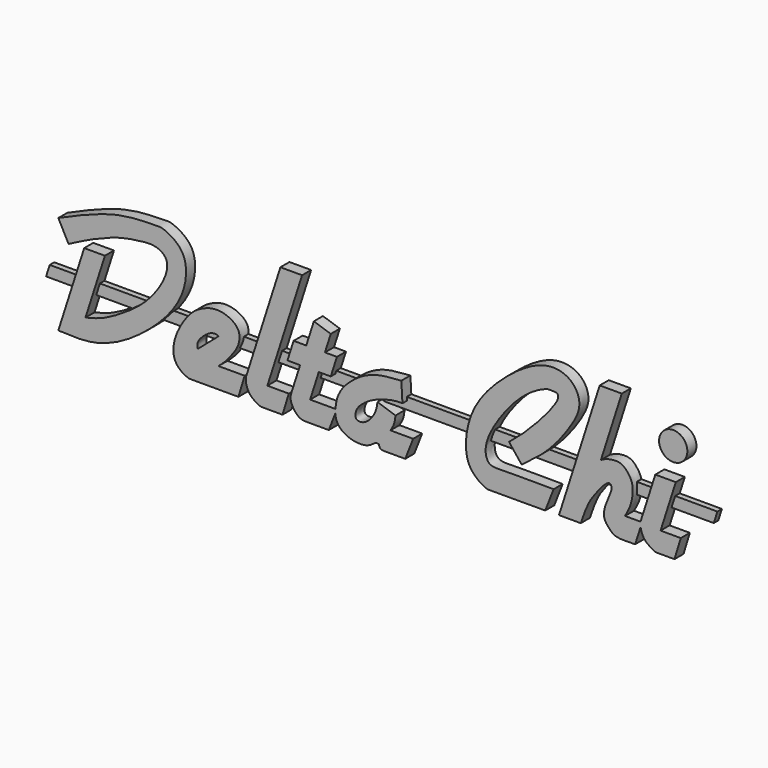
from build123d import *

# Parameters (mm, degrees)
F1_DEPTH = 1.27
F0_R     = 1.5843769343
F4_DEPTH = 0.635
F5_DEPTH = 0.635


with BuildPart() as f1:
    # F0 (on Front) → F1 (new body)
    with BuildSketch(Plane.XZ):
        with BuildLine():
            Line((11.5583368814, 2.9581922572), (9.238501317, 2.9581922572))
            Line((9.238501317, 2.9581922572), (6.3397404738, -6.112227682))
            add(Edge.make_bspline(
                [(6.3397404738, -6.112227682), (7.4441484176, -6.1544100754), (11.509628416, -6.5846275927), (17.9109968749, -1.8961025658), (20.4928464292, 1.9472420269), (20.817384408, 5.0494202074), (19.9129921351, 6.8743066297), (17.9478352073, 7.8694620029), (17.2190347579, 7.7492274241), (12.7951441267, 7.8669975564), (8.7299015863, 6.0410147356), (6.3397404738, 4.9838235872)],
                knots=[0, 0, 0, 0, 0.1269238793, 0.2901043112, 0.4152988438, 0.5132554474, 0.5948026218, 0.6765960194, 0.7255936362, 0.8411976173, 1, 1, 1, 1], degree=3))
            Line((6.3397404738, 4.9838235872), (7.4859545566, 2.7952580713))
            add(Edge.make_bspline(
                [(7.4859545566, 2.7952580713), (8.2236601536, 3.1805826506), (9.8172231795, 4.01295741), (12.9982791172, 5.3295282857), (15.1573844049, 5.6487607974), (17.2331239985, 5.9184782824), (18.7492748451, 4.9172200411), (18.3797124669, 2.7652905985), (16.3268092986, -0.1702231309), (13.6664187703, -2.0050802173), (11.597224487, -3.2305518663), (10.2401798172, -3.6615941397), (9.3834213912, -3.8472663146)],
                knots=[0, 0, 0, 0, 0.1035319794, 0.2210262779, 0.3162776823, 0.4065161292, 0.4835580268, 0.5705705005, 0.6913426498, 0.8065191141, 0.9033937832, 1, 1, 1, 1], degree=3))
            Line((9.3834213912, -3.8472663146), (11.5583368814, 2.9581922572))
        make_face()
    extrude(amount=F1_DEPTH)


with BuildPart() as f1b:
    # F0 (on Front) → F1, piece 2 (new body)
    with BuildSketch(Plane.XZ):
        with BuildLine():
            Line((27.2133555263, -3.7849494256), (24.2806579918, -3.7849494256))
            add(Edge.make_bspline(
                [(20.934375003, -6.0972687788), (20.6237746916, -5.9553557041), (19.9688638955, -5.656127399), (19.0898046825, -4.5438356782), (19.3260874159, -2.3470660746), (20.6114467926, -0.1690673469), (21.7037779099, 0.9830999374), (23.5887847531, 1.8522113729), (25.3229288137, 1.5984111399), (26.7458523187, 0.6140665528), (26.6181462164, -1.0302522959), (25.8346105799, -2.1262963733), (25.1208132675, -3.0535019221), (24.5582846254, -3.5432449289), (24.2806579918, -3.7849494256)],
                knots=[0, 0, 0, 0, 0.0683310471, 0.1440782214, 0.2416800374, 0.3481729944, 0.4329900458, 0.5268903062, 0.6150450793, 0.6982655618, 0.7790626002, 0.8570259985, 0.929437565, 1, 1, 1, 1], degree=3))
            Line((20.934375003, -6.0972687788), (26.5177804977, -6.0972687788))
            Line((26.5177804977, -6.0972687788), (27.2133555263, -3.7849494256))
        make_face()
        with BuildLine():
            add(Edge.make_bspline(
                [(21.9683405012, -2.8449825477), (22.739112998, -2.1807390925), (23.5098854949, -1.5164956373), (24.2806579918, -0.8522521821)],
                knots=[0, 0, 0, 0, 3.0525049529, 3.0525049529, 3.0525049529, 3.0525049529], degree=3))
            add(Edge.make_bspline(
                [(21.9683405012, -2.8449825477), (21.9220461308, -2.6323953166), (21.8022425221, -2.1277051513), (22.9283600883, -1.0010714427), (23.7222803055, -0.6785461743), (24.1428096339, -0.7291242349), (24.2806579918, -0.8522521821)],
                knots=[0, 0, 0, 0, 0.2196054864, 0.550181783, 0.8035281405, 1, 1, 1, 1], degree=3))
        make_face(mode=Mode.SUBTRACT)
    extrude(amount=F1_DEPTH)


with BuildPart() as f1c:
    # F0 (on Front) → F1, piece 3 (new body)
    with BuildSketch(Plane.XZ):
        with BuildLine():
            Line((29.7624055112, -3.9401776428), (33.6480308079, 8.2182083279))
            Line((33.6480308079, 8.2182083279), (31.2219001353, 8.2182083279))
            Line((31.2219001353, 8.2182083279), (27.395882284, -3.7536618897))
            add(Edge.make_bspline(
                [(27.395882284, -3.7536618897), (27.3626673092, -3.9107859252), (27.2830365237, -4.2882497343), (27.6099014615, -5.2582507547), (28.1522354832, -5.7998826823), (28.6683587416, -6.0880579287), (28.9955866819, -6.2549276858), (29.1592962131, -6.2536320454)],
                knots=[0, 0, 0, 0, 0.1777965485, 0.4222191522, 0.6373839909, 0.8255478489, 1, 1, 1, 1], degree=3))
            Line((29.1592962131, -6.2536320454), (31.4544699177, -6.2536320454))
            Line((31.4544699177, -6.2536320454), (32.1586950704, -3.9401776428))
            Line((32.1586950704, -3.9401776428), (29.7624055112, -3.9401776428))
        make_face()
    extrude(amount=F1_DEPTH)


with BuildPart() as f1d:
    # F0 (on Front) → F1, piece 4 (new body)
    with BuildSketch(Plane.XZ):
        with BuildLine():
            Line((34.1174524835, 1.4392599511), (32.6996871635, 1.4392599511))
            Line((32.6996871635, 1.4392599511), (32.0095790109, -0.7201354202))
            Line((32.0095790109, -0.7201354202), (33.427344331, -0.7201354202))
            Line((33.427344331, -0.7201354202), (32.3894061148, -3.9679147303))
            add(Edge.make_bspline(
                [(32.3894061148, -3.9679147303), (32.3539821517, -4.2074069235), (32.3077429237, -4.5448398513), (32.8789397145, -5.6686856111), (33.6315587034, -6.0905655252), (34.0119533579, -6.0804787938), (34.1916170495, -6.0811438617)],
                knots=[0, 0, 0, 0, 0.2197878812, 0.5298954364, 0.7910428436, 1, 1, 1, 1], degree=3))
            Line((34.1916170495, -6.0811438617), (36.6396096127, -6.0811438617))
            Line((36.6396096127, -6.0811438617), (37.3817411468, -4.1773119798))
            add(Edge.make_bspline(
                [(37.390926157, -3.7552919632), (37.3804727481, -3.896675323), (37.3761926951, -4.0379928618), (37.3817411468, -4.1773119798)],
                knots=[0.5705734468, 0.5705734468, 0.5705734468, 0.5705734468, 0.6009630692, 0.6009630692, 0.6009630692, 0.6009630692], degree=3))
            Line((37.390926157, -3.7552919632), (34.5505749426, -3.7552919632))
            Line((34.5505749426, -3.7552919632), (35.5205623301, -0.7201354202))
            Line((35.5205623301, -0.7201354202), (36.8627270243, -0.7201354202))
            Line((36.8627270243, -0.7201354202), (37.5528351768, 1.4392599511))
            Line((37.5528351768, 1.4392599511), (36.2106704826, 1.4392599511))
            Line((36.2106704826, 1.4392599511), (36.8627270243, 3.4795892425))
            Line((36.8627270243, 3.4795892425), (34.9704111173, 4.10822556))
            Line((34.9704111173, 4.10822556), (34.1174524835, 1.4392599511))
        make_face()
        with BuildLine():
            add(Edge.make_bspline(
                [(37.390926157, -3.7552919632), (37.3804727481, -3.896675323), (37.3761926951, -4.0379928618), (37.3817411468, -4.1773119798)],
                knots=[0.5705734468, 0.5705734468, 0.5705734468, 0.5705734468, 0.6009630692, 0.6009630692, 0.6009630692, 0.6009630692], degree=3))
            add(Edge.make_bspline(
                [(37.3817411468, -4.1773119798), (37.392328196, -4.4431480099), (37.5312347254, -5.2176693669), (38.7220219736, -6.236897387), (40.8587848965, -6.4300522573), (41.5571529811, -5.8736297488), (41.8619178236, -5.6308093481)],
                knots=[0.6009630692, 0.6009630692, 0.6009630692, 0.6009630692, 0.6589497741, 0.7746633228, 0.9016640387, 1, 1, 1, 1], degree=3))
            Line((41.8619178236, -5.6308093481), (42.2533527017, -5.6308093481))
            add(Edge.make_bspline(
                [(42.2533527017, -5.6308093481), (42.2675923832, -5.7180727897), (42.2968327159, -5.8972630384), (42.4875444347, -6.1218789339), (42.8100095232, -6.1339937311), (42.8472571075, -6.1338087544)],
                knots=[0, 0, 0, 0, 0.2963318136, 0.608499623, 0.9364444921, 0.9364444921, 0.9364444921, 0.9364444921], degree=3))
            Line((42.8472571075, -6.1338087544), (45.2066808939, -6.1332210898))
            Line((45.2066808939, -6.1332210898), (46.0903713247, -3.8662401858))
            Line((46.0903713247, -3.8662401858), (43.5422138314, -3.8662401858))
            add(Edge.make_bspline(
                [(43.5422138314, -3.8662401858), (43.6434718788, -3.7248078476), (43.955566276, -3.202149882), (44.0373991751, -2.8050103574), (44.1166646779, -2.2105039097)],
                knots=[0, 0, 0, 0, 0.4355065819, 1, 1, 1, 1], degree=3))
            Line((44.1166646779, -2.2105039097), (42.0921580655, -1.5379532131))
            add(Edge.make_bspline(
                [(44.8928326368, -0.7567268331), (44.4289408624, -0.7455486339), (44.334726943, -0.7630375022), (43.4964447415, -0.834955831), (41.5388628103, -1.390907753), (40.090989198, -2.4696041182), (39.6410756327, -3.1901824428), (39.5414913588, -4.1442095313), (40.8415428068, -4.1903256763), (41.961217304, -2.6601737366), (42.0533731488, -1.8780982635), (42.0921580655, -1.5379532131)],
                knots=[0, 0, 0, 0, 0.0840952071, 0.1697088013, 0.3216193436, 0.4624728163, 0.5586747749, 0.6467834882, 0.7479812036, 0.8890732838, 1, 1, 1, 1], degree=3))
            Line((44.8928326368, -0.7567268331), (44.7697676718, 1.432727091))
            add(Edge.make_bspline(
                [(44.7697676718, 1.432727091), (43.7008223192, 1.3640593706), (41.648313579, 1.232208761), (39.3385119054, -0.1260462045), (37.7342234004, -1.8446619748), (37.4613840971, -3.0431148695), (37.3978194533, -3.6620594683), (37.390926157, -3.7552919632)],
                knots=[0, 0, 0, 0, 0.1578260616, 0.3030457732, 0.4375753345, 0.5505336039, 0.5705734468, 0.5705734468, 0.5705734468, 0.5705734468], degree=3))
        make_face()
    extrude(amount=F1_DEPTH)


with BuildPart() as f1e:
    # F0 (on Front) → F1, piece 5 (new body)
    with BuildSketch(Plane.XZ):
        with BuildLine():
            add(Edge.make_bspline(
                [(56.8344220519, -0.6727006403), (57.536092901, -0.0985210669), (58.981812623, 1.0845161568), (61.4522683866, 3.8814649904), (61.4833894251, 4.0843152011), (62.367054076, 5.1445088036), (62.3973875748, 5.9770064502), (61.5374535241, 5.9113985648), (61.1907722065, 6.0054789768), (59.3549616868, 5.219553597), (56.8962905087, 3.0575959186), (54.476325238, -0.5239799869), (54.0840321515, -2.5259321439), (54.5585012014, -3.7841258338), (56.4829070286, -3.6899333482), (59.7177449421, -3.7098362799), (61.8280459066, -3.723213362)],
                knots=[0, 0, 0, 0, 0.0930582141, 0.1917435104, 0.2179368983, 0.2792954818, 0.3217037626, 0.3653724828, 0.397525177, 0.4677311533, 0.5674134201, 0.678450431, 0.7529723589, 0.8065968651, 0.873879835, 1, 1, 1, 1], degree=3))
            Line((56.8344220519, -0.6727006403), (58.2509338856, -2.4686302058))
            add(Edge.make_bspline(
                [(58.2509338856, -2.4686302058), (58.4671273828, -2.2947364487), (58.653230403, -2.0939955812), (61.2401562782, -0.3340070928), (63.8132491254, 3.0521447417), (65.1156690008, 5.6462437526), (63.8351395983, 8.0752841997), (60.2374798056, 8.7326906295), (54.9538299971, 4.5474881989), (52.5011949099, 1.0432474754), (51.8172413088, -2.415022098), (52.3018042793, -4.9135195574), (54.0605011917, -6.0731752268), (54.5331237261, -6.1424866279), (54.5733683978, -6.1474639068), (60.2808153305, -6.1354543984), (60.8894621988, -6.1310150856)],
                knots=[0, 0, 0, 0, 0.0338861178, 0.1086849092, 0.2033726715, 0.2762020347, 0.3423872005, 0.4207228438, 0.5341164091, 0.6272992911, 0.7084751446, 0.7780444737, 0.8398677078, 0.866251273, 0.8837492923, 0.9909216554, 0.9909216554, 0.9909216554, 0.9909216554], degree=3))
            Line((60.8894621988, -6.1310150856), (61.8280459066, -3.723213362))
        make_face()
    extrude(amount=F1_DEPTH)


with BuildPart() as f1f:
    # F0 (on Front) → F1, piece 6 (new body)
    with BuildSketch(Plane.XZ):
        with BuildLine():
            Line((66.9940567642, 8.1950222574), (62.4304637313, -6.0847708955))
            Line((62.4304637313, -6.0847708955), (64.8716390133, -6.0847708955))
            add(Edge.make_bspline(
                [(64.8716390133, -6.0847708955), (64.9763642646, -5.7314444494), (65.3113821699, -4.8136837528), (65.8788110997, -3.4582361982), (66.6711638205, -2.4563300411), (67.2341715854, -1.6631813625), (68.1666941651, -0.8457293994), (68.449894567, -1.6855497607), (67.7251359557, -2.9881592018), (67.2711232708, -4.6517195726), (68.0296074984, -5.5527121429), (68.7566935376, -6.2902897156), (70.0967212544, -6.1977129943), (70.9676982654, -6.1819385307)],
                knots=[0, 0, 0, 0, 0.0940386819, 0.1947266023, 0.286033855, 0.3709752136, 0.4506078612, 0.508931595, 0.6105547438, 0.7159243693, 0.7998688722, 0.8786044105, 1, 1, 1, 1], degree=3))
            Line((70.9676982654, -6.1819385307), (71.5720379679, -4.2909184761))
            add(Edge.make_bspline(
                [(71.5710121124, -3.7578128137), (71.5441535969, -3.8975253136), (71.5336089809, -4.0521583348), (71.5670617144, -4.2631440018), (71.5720379679, -4.2909184761)],
                knots=[0.0137477144, 0.0137477144, 0.0137477144, 0.0137477144, 0.1731956127, 0.1966109127, 0.1966109127, 0.1966109127, 0.1966109127], degree=3))
            Line((71.5710121124, -3.7578128137), (69.8300384912, -3.7578128137))
            add(Edge.make_bspline(
                [(67.1309805195, 0.8867597493), (67.3340182593, 0.9992655484), (67.8150259898, 1.2657686397), (69.369655112, 1.4777996976), (70.1951225015, 0.6081433229), (70.8397112827, -0.4415409908), (70.5571540861, -2.5072653543), (70.0498844289, -3.3604386206), (69.8300384912, -3.7578128137)],
                knots=[0, 0, 0, 0, 0.1288060496, 0.3049437453, 0.4582521101, 0.6175575441, 0.8236651085, 1, 1, 1, 1], degree=3))
            Line((67.1309805195, 0.8867597493), (69.4665840894, 8.1950222574))
            Line((69.4665840894, 8.1950222574), (66.9940567642, 8.1950222574))
        make_face()
        with BuildLine():
            add(Edge.make_bspline(
                [(71.5710121124, -3.7578128137), (71.5441535969, -3.8975253136), (71.5336089809, -4.0521583348), (71.5670617144, -4.2631440018), (71.5720379679, -4.2909184761)],
                knots=[0.0137477144, 0.0137477144, 0.0137477144, 0.0137477144, 0.1731956127, 0.1966109127, 0.1966109127, 0.1966109127, 0.1966109127], degree=3))
            add(Edge.make_bspline(
                [(71.5720379679, -4.2909184761), (71.6194594312, -4.5555967542), (71.8370975302, -5.2135369306), (72.3605804566, -5.7393451035), (72.8886416365, -6.003119047), (73.1790271773, -6.2227930925), (73.341757151, -6.2215052046)],
                knots=[0.1966109127, 0.1966109127, 0.1966109127, 0.1966109127, 0.4197482157, 0.6367880894, 0.8265916848, 1, 1, 1, 1], degree=3))
            Line((73.341757151, -6.2215052046), (75.3721089563, -6.2215052046))
            Line((75.3721089563, -6.2215052046), (76.076334109, -3.908050802))
            Line((76.076334109, -3.908050802), (73.8132742946, -3.908050802))
            Line((73.8132742946, -3.908050802), (75.5176777163, 1.4251434891))
            Line((75.5176777163, 1.4251434891), (73.2231391982, 1.4251434891))
            Line((73.2231391982, 1.4251434891), (71.578343222, -3.7215350489))
            add(Edge.make_bspline(
                [(71.578343222, -3.7215350489), (71.5757749495, -3.7336843082), (71.5733278733, -3.7457666998), (71.5710121124, -3.7578128137)],
                knots=[0, 0, 0, 0, 0.0137477144, 0.0137477144, 0.0137477144, 0.0137477144], degree=3))
        make_face()
    extrude(amount=F1_DEPTH)


with BuildPart() as f1g:
    # F0 (on Front) → F1, piece 7 (new body)
    with BuildSketch(Plane.XZ):
        with Locations((75.2293908452, 4.8940147229)):
            Circle(F0_R)
    extrude(amount=F1_DEPTH)


with BuildPart() as f1_1:
    # F2: moved
    add(f1.part.moved(Location((0, 0, 1.016))))



with BuildPart() as f1b_1:
    # F2: moved
    add(f1b.part.moved(Location((0, 0, 1.016))))


with BuildPart() as f1c_1:
    # F2: moved
    add(f1c.part.moved(Location((0, 0, 1.016))))


with BuildPart() as f1d_1:
    # F2: moved
    add(f1d.part.moved(Location((0, 0, 1.016))))


with BuildPart() as f1e_1:
    # F2: moved
    add(f1e.part.moved(Location((0, 0, 1.016))))


with BuildPart() as f1f_1:
    # F2: moved
    add(f1f.part.moved(Location((0, 0, 1.016))))


with BuildPart() as f1g_1:
    # F2: moved
    add(f1g.part.moved(Location((0, 0, 1.016))))


with BuildPart() as f1_2:
    add(f1_1.part)

    add(f1b_1.part)  # F4 merges F1b

    add(f1c_1.part)  # F4 merges F1c

    add(f1d_1.part)  # F4 merges F1d

    add(f1e_1.part)  # F4 merges F1e

    add(f1f_1.part)  # F4 merges F1f
    # F3 (on Front) → F4 (join)
    with BuildSketch(Plane.XZ):
        Polygon((79.6712024446, 0.635), (4.8660361676, 0.635), (4.4601645216, -0.635), (79.2653307985, -0.635), align=None)
    extrude(amount=F4_DEPTH)


with BuildPart() as f5:
    # F0 (on Front) → F5 (new body)
    with BuildSketch(Plane.XZ):
        with BuildLine():
            add(Edge.make_bspline(
                [(16.4142258787, -11.0682983595), (50.9742268626, -16.8183967536), (77.3812885674, -8.4572114996), (103.7883502723, -0.0960262456), (77.7293858456, 8.3457287327)],
                knots=[1.0222549469, 1.0222549469, 1.0222549469, 2.4313865711, 2.4313865711, 3.8405181954, 3.8405181954, 3.8405181954], degree=2, weights=[1, 0.7618928484, 1, 0.7618928484, 1]))
            add(Edge.make_bspline(
                [(16.4142258787, -11.0682983595), (13.3993673343, -10.5666857211), (8.3808144511, -10.1248051011), (-0.1767272457, -6.1655253178), (-2.1760582318, -3.4980937313), (-3.3019293041, -1.2062395478), (-3.3365795401, -0.2624513976), (-3.3536800183, 0)],
                knots=[0, 0, 0, 0, 0.2825195318, 0.5717051514, 0.7474505389, 0.8984687445, 1, 1, 1, 1], degree=3))
            Line((-3.3536800183, 0), (-5.4217712022, 0))
            add(Edge.make_bspline(
                [(-5.4217712022, 0), (-5.4615566787, -0.8868223517), (-4.9461295133, -3.0305590008), (-2.2075652853, -6.8205672735), (2.1033537416, -9.3382774884), (7.484946702, -11.7437297194), (13.5745781312, -12.7029469698), (16.174225298, -13.3736926873)],
                knots=[0, 0, 0, 0, 0.1490333784, 0.3351226406, 0.5278361037, 0.7411327195, 1, 1, 1, 1], degree=3))
            add(Edge.make_bspline(
                [(16.174225298, -13.3736926873), (117.5996857499, -31.3687014148), (90.0391311221, 3.6079933972), (62.4785764943, 38.5846882092), (-0.9252044806, 8.326942329)],
                knots=[1.0471539652, 1.0471539652, 1.0471539652, 3.3791414734, 3.3791414734, 5.7111289817, 5.7111289817, 5.7111289817], degree=2, weights=[1, 0.3938372967, 1, 0.3938372967, 1]))
            Line((-0.9252044806, 8.326942329), (0.030855203, 6.5014550262))
            add(Edge.make_bspline(
                [(77.7293858456, 8.3457287327), (34.054378504, 22.4941693467), (0.030855203, 6.5014550262)],
                knots=[3.8405181954, 3.8405181954, 3.8405181954, 5.7581826357, 5.7581826357, 5.7581826357], degree=2, weights=[1, 0.5744762302, 1]))
        make_face()
    extrude(amount=F5_DEPTH)


with BuildPart() as f5_1:
    # F6: moved
    add(f5.part.moved(Location((0, 0, 2.032))))


solid = Compound([f1g_1.part, f1_2.part])
